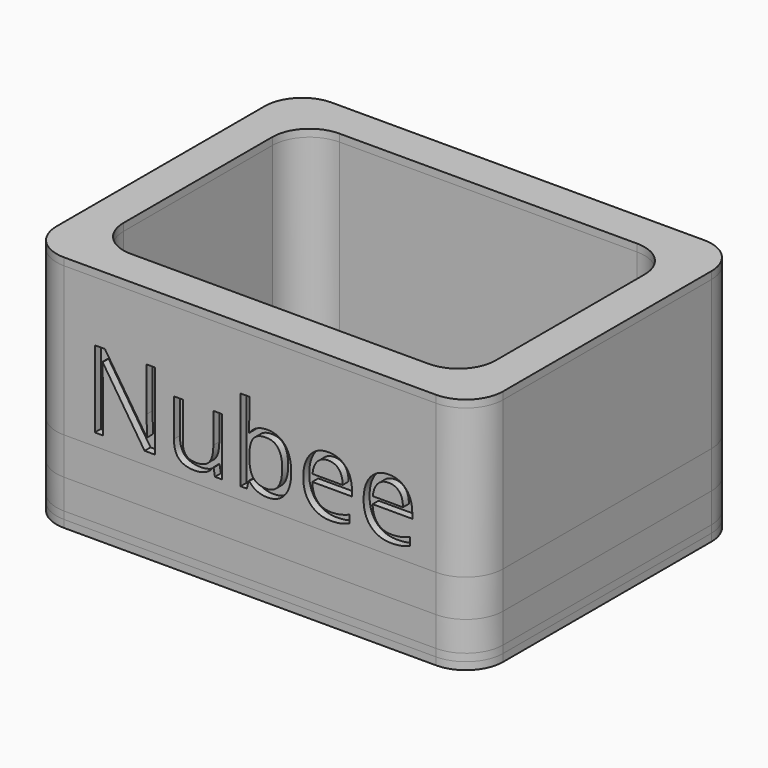
from build123d import *

# Parameters (mm, degrees)
F0_W         = 60
F0_H         = 45
F0_W_2       = 50
F0_H_2       = 35
F1_DEPTH     = 12.5
F2_R         = 5
F3_R         = 5
F4_DEPTH     = 5
F5_DEPTH     = 1
F7_DEPTH     = 1
F8_TEXT_SIZE = 14.4455033355
F9_DEPTH     = 1


# Not quite as in the source:
# - Text() gives the source's letters only with a copy of the font that has no kerning and outlines rounded to 1/6400 em; it was checked with that copy


with BuildPart() as f1:
    # F0 (on Top) → F1 (new body, symmetric)
    with BuildSketch(Plane.XY):
        Rectangle(F0_W, F0_H)
        Rectangle(F0_W_2, F0_H_2, mode=Mode.SUBTRACT)
    extrude(amount=F1_DEPTH, both=True)

    # F2
    f2_edges = [f1.edges().sort_by_distance(p)[0] for p in [
        (-25, 17.5, 0),
        (-25, -17.5, 0),
        (25, -17.5, 0),
    ]]
    fillet(f2_edges, radius=F2_R)

    # F3
    f3_edges = [f1.edges().sort_by_distance(p)[0] for p in [
        (25, 17.5, 0),
        (30, -22.5, 0),
        (-30, -22.5, 0),
        (-30, 22.5, 0),
        (30, 22.5, 0),
    ]]
    fillet(f3_edges, radius=F3_R)

    # F4 (add, symmetric): a face of the model
    f4_faces = [f1.faces().sort_by_distance(p)[0] for p in [
        (25.75, 0, -12.5),
    ]]
    extrude(f4_faces, amount=F4_DEPTH, both=True)

    # F5 (add, symmetric): a face of the model
    f5_faces = [f1.faces().sort_by_distance(p)[0] for p in [
        (25.75, 0, -17.5),
    ]]
    extrude(f5_faces, amount=F5_DEPTH, both=True)

    # F7 (add): a face of the model
    f7_faces = [f1.faces().sort_by_distance(p)[0] for p in [
        (25.75, 0, 12.5),
    ]]
    extrude(f7_faces, amount=F7_DEPTH)

    # F8 (on face) → F9 (cut)
    with BuildSketch(Plane.XZ.offset(22.5)):
        with Locations((-22.2653661878, -5.8611472664)):
            Text('Nubee', F8_TEXT_SIZE, font='Open Sans', text_align=(TextAlign.LEFT, TextAlign.BOTTOM))
    extrude(amount=-F9_DEPTH, mode=Mode.SUBTRACT)


solid = f1.part
